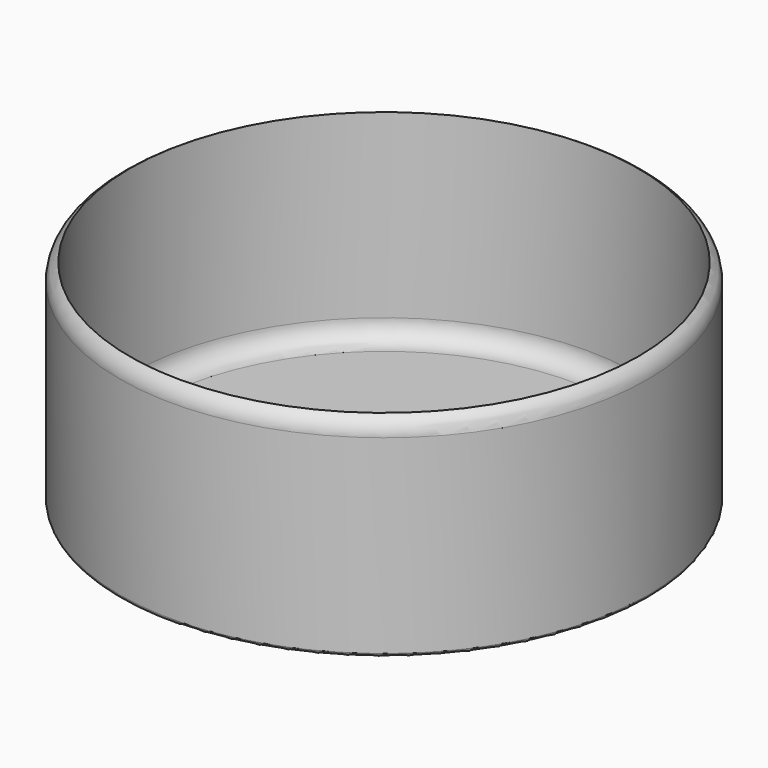
from build123d import *

# Parameters (mm, degrees)
F0_R     = 68.9281560168
F1_DEPTH = 54.864
F2_T     = -2.54
F4_R     = 0.9
F5_R     = 5.08


# Not quite as in the source:
# - a fillet or chamfer that OpenCascade refuses, or shapes differently, is made with other operations: its cross-section is extruded or revolved along the edge and cut away or added


with BuildPart() as f1:
    # F0 (on Top) → F1 (new body)
    with BuildSketch(Plane.XY):
        Circle(F0_R)
    extrude(amount=F1_DEPTH)

    # F2
    f2_openings = [f1.faces().sort_by_distance(p)[0] for p in [
        (0, 0, 54.864),
    ]]
    offset(amount=F2_T, openings=f2_openings)

    # F3: fillet of radius 5.08 on 1 edges, made by hand

    # F3_s1 → F3_t2 (revolve, cut)
    with BuildSketch(Plane.XZ):
        with BuildLine():
            ThreePointArc((68.9281560168, 50.4645909488), (68.247565068, 53.0045909488), (66.3881560168, 54.864))
            Line((66.3881560168, 54.864), (68.9281560168, 54.864))
            Line((68.9281560168, 54.864), (68.9281560168, 50.4645909488))
        make_face()
    revolve(axis=Axis((0, 0, 54.864), (0, 0, 1)), mode=Mode.SUBTRACT)

    # F4
    f4_edges = [f1.edges().sort_by_distance(p)[0] for p in [
        (-68.928156, 0, 0),
    ]]
    fillet(f4_edges, radius=F4_R)

    # F5
    f5_edges = [f1.edges().sort_by_distance(p)[0] for p in [
        (-66.388156, 0, 2.54),
    ]]
    fillet(f5_edges, radius=F5_R)


solid = f1.part
